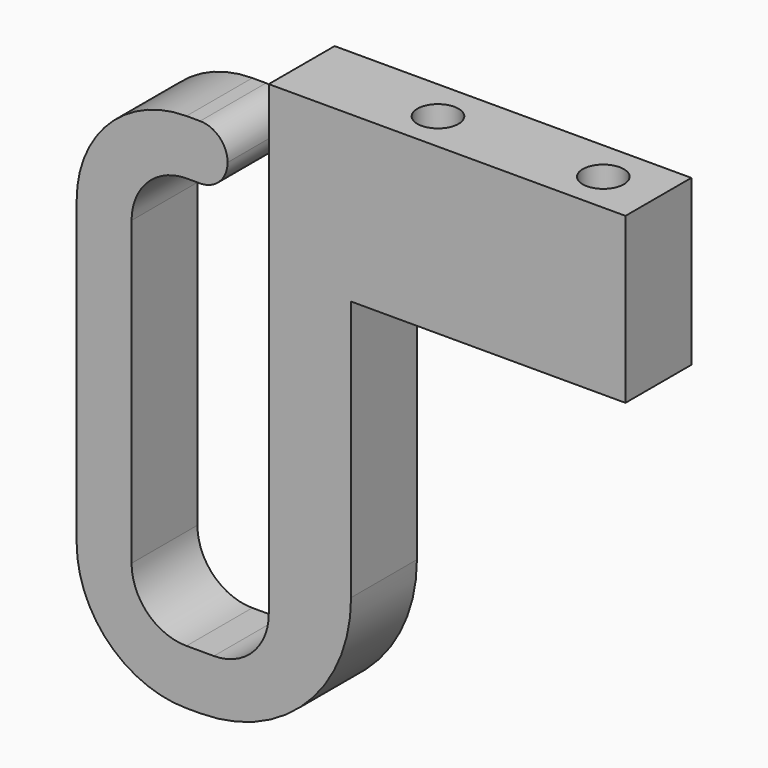
from build123d import *

# Parameters (mm, degrees)
F1_DEPTH       = 6
F2_R           = 4
F3_R           = 8
F4_R           = 11
F5_R           = 1.99999
F7_D           = 3
F7_CSINK_D     = 5
F7_CSINK_ANGLE = 90


# Not quite as in the source:
# - a fillet or chamfer is up to 0.001 mm smaller than in the source, because OpenCascade refuses the exact size


with BuildPart() as f1:
    # F0 (on Front) → F1 (new body)
    with BuildSketch(Plane.XZ):
        Polygon((0, 0), (0, 30), (7, 30), (7, 34), (-4, 34), (-4, -4), (16, -4), (16, 26), (36, 26), (36, 38), (10, 38), (10, 0), align=None)
    extrude(amount=F1_DEPTH)

    # F2
    f2_edges = [f1.edges().sort_by_distance(p)[0] for p in [
        (10, -3, 0),
        (0, -3, 0),
        (0, -3, 30),
    ]]
    fillet(f2_edges, radius=F2_R)

    # F3
    f3_edges = [f1.edges().sort_by_distance(p)[0] for p in [
        (-4, -3, 34),
        (-4, -3, -4),
    ]]
    fillet(f3_edges, radius=F3_R)

    # F4
    f4_edges = [f1.edges().sort_by_distance(p)[0] for p in [
        (16, -3, -4),
    ]]
    fillet(f4_edges, radius=F4_R)

    # F5 (radius 2 in the source; OpenCascade refuses exactly that, so slightly less here)
    f5_edges = [f1.edges().sort_by_distance(p)[0] for p in [
        (7, -3, 34),
        (7, -3, 30),
    ]]
    fillet(f5_edges, radius=F5_R)

    # F7 (through all)
    with Locations(Plane(origin=(0, 0, 26), x_dir=(1, 0, 0), z_dir=(0, 0, -1))):
        with Locations((20, 3.0815127769), (31.9998442765, 3.0203789876)):
            CounterSinkHole(F7_D / 2, F7_CSINK_D / 2, counter_sink_angle=F7_CSINK_ANGLE)


solid = f1.part
